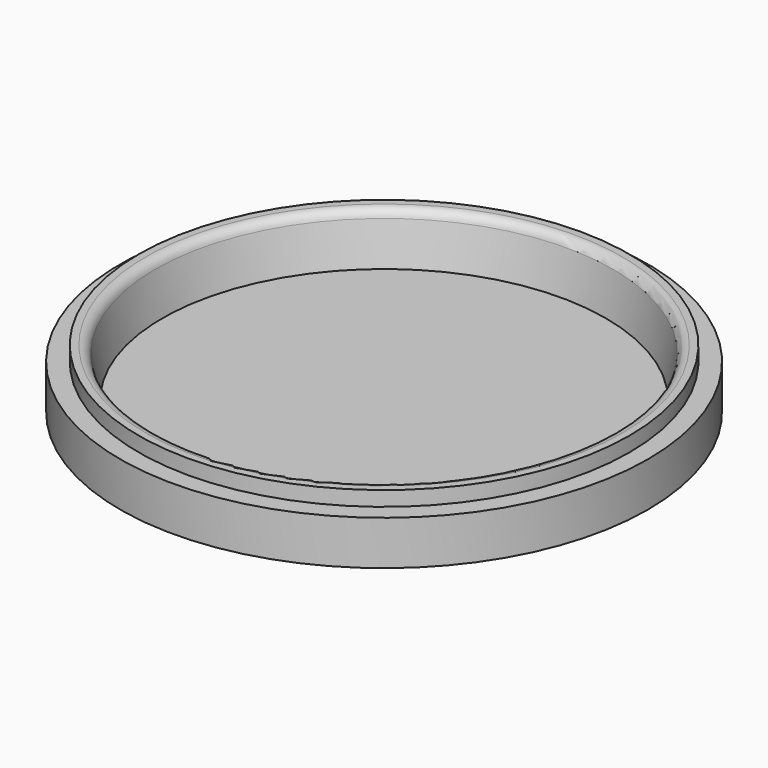
from build123d import *

# Parameters (mm, degrees)
F0_R     = 25
F1_DEPTH = 1
F5_R     = 25
F5_R_2   = 23.25
F6_DEPTH = 3.2
F7_R     = 0.9


with BuildPart() as f1:
    # F0 (on Top) → F1 (new body)
    with BuildSketch(Plane.XY):
        Circle(F0_R)
    extrude(amount=F1_DEPTH)

    # F3 (on Front) → F4 (revolve)
    with BuildSketch(Plane.XZ):
        Polygon((21, 1), (23.25, 1), (23.25, 5.6), (21.8255799264, 5.6), align=None)
    revolve(axis=Axis((0, 0, 1), (0, 0, 1)))

    # F5 (on face) → F6 (join)
    with BuildSketch(Plane.XY.offset(1)):
        Circle(F5_R)
        Circle(F5_R_2, mode=Mode.SUBTRACT)
    extrude(amount=F6_DEPTH)

    # F7
    f7_edges = [f1.edges().sort_by_distance(p)[0] for p in [
        (-21.82558, 0, 5.6),
    ]]
    fillet(f7_edges, radius=F7_R)


solid = f1.part
